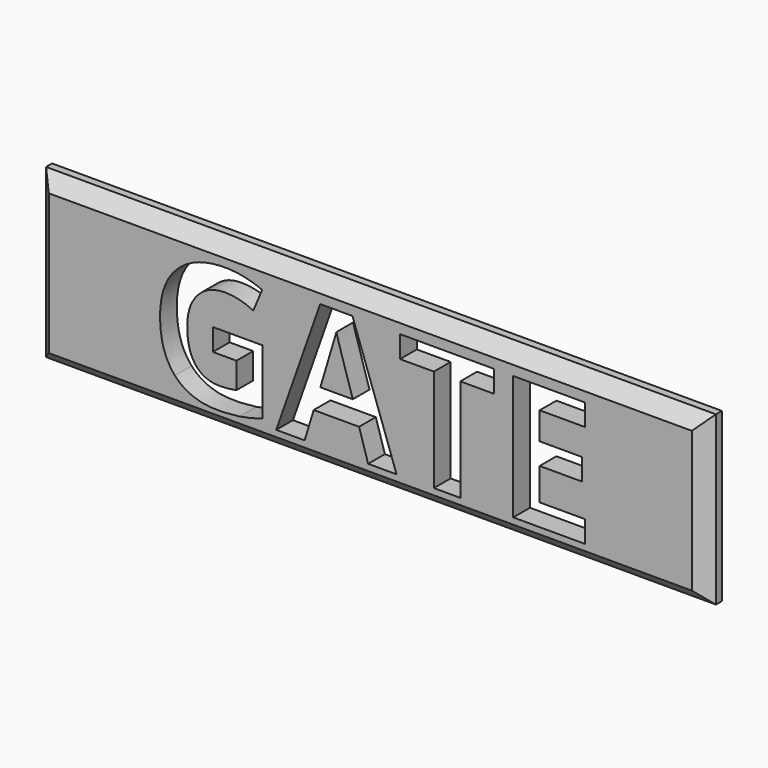
from build123d import *

# Parameters (mm, degrees)
F0_W     = 50.8
F0_H     = 12.7
F1_DEPTH = 1.5875
F2_SIZE  = 1.016


# Not quite as in the source:
# - a feature names something its author has since deleted; it is built from what else it names


with BuildPart() as f1:
    # F0 (on Front) → F1 (new body)
    with BuildSketch(Plane.XZ):
        with Locations((-9.1615320603, 10.3311909613)):
            Rectangle(F0_W, F0_H)
        with BuildLine():
            Line((-21.1010067493, 9.1154048977), (-21.1010067493, 10.7835201321))
            Line((-21.1010067493, 10.7835201321), (-17.3534318796, 10.7835201321))
            Line((-17.3534318796, 10.7835201321), (-17.3534318796, 5.8866614081))
            add(Edge.make_bspline(
                [(-17.3534318796, 5.8866614081), (-18.2650041452, 5.5890051581), (-19.0690894316, 5.4691158352)],
                knots=[0, 0, 0, 1, 1, 1], degree=2))
            add(Edge.make_bspline(
                [(-19.0690894316, 5.4691158352), (-19.8731747181, 5.3492265123), (-20.7123999785, 5.3492265123)],
                knots=[0, 0, 0, 1, 1, 1], degree=2))
            add(Edge.make_bspline(
                [(-20.7123999785, 5.3492265123), (-22.8497372181, 5.3492265123), (-23.9773169707, 6.6059973456)],
                knots=[0, 0, 0, 1, 1, 1], degree=2))
            add(Edge.make_bspline(
                [(-23.9773169707, 6.6059973456), (-25.1048967233, 7.862768179), (-25.1048967233, 10.2150793769)],
                knots=[0, 0, 0, 1, 1, 1], degree=2))
            add(Edge.make_bspline(
                [(-25.1048967233, 10.2150793769), (-25.1048967233, 12.5012447415), (-23.7964494577, 13.7797196764)],
                knots=[0, 0, 0, 1, 1, 1], degree=2))
            add(Edge.make_bspline(
                [(-23.7964494577, 13.7797196764), (-22.4880021921, 15.0581946113), (-20.1708309681, 15.0581946113)],
                knots=[0, 0, 0, 1, 1, 1], degree=2))
            add(Edge.make_bspline(
                [(-20.1708309681, 15.0581946113), (-18.7156226348, 15.0581946113), (-17.3658342233, 14.4773515123)],
                knots=[0, 0, 0, 1, 1, 1], degree=2))
            Line((-17.3658342233, 14.4773515123), (-18.0314266712, 12.8753821113))
            add(Edge.make_bspline(
                [(-18.0314266712, 12.8753821113), (-19.0649553171, 13.3921464342), (-20.1832333118, 13.3921464342)],
                knots=[0, 0, 0, 1, 1, 1], degree=2))
            add(Edge.make_bspline(
                [(-20.1832333118, 13.3921464342), (-21.481345291, 13.3921464342), (-22.2626929473, 12.5198482571)],
                knots=[0, 0, 0, 1, 1, 1], degree=2))
            add(Edge.make_bspline(
                [(-22.2626929473, 12.5198482571), (-23.0440406035, 11.64755008), (-23.0440406035, 10.1758052883)],
                knots=[0, 0, 0, 1, 1, 1], degree=2))
            add(Edge.make_bspline(
                [(-23.0440406035, 10.1758052883), (-23.0440406035, 8.6379146633), (-22.4146216582, 7.827628205)],
                knots=[0, 0, 0, 1, 1, 1], degree=2))
            add(Edge.make_bspline(
                [(-22.4146216582, 7.827628205), (-21.7852027129, 7.0173417467), (-20.5842424264, 7.0173417467)],
                knots=[0, 0, 0, 1, 1, 1], degree=2))
            add(Edge.make_bspline(
                [(-20.5842424264, 7.0173417467), (-19.9558570098, 7.0173417467), (-19.3109351348, 7.1454992988)],
                knots=[0, 0, 0, 1, 1, 1], degree=2))
            Line((-19.3109351348, 7.1454992988), (-19.3109351348, 9.1154048977))
            Line((-19.3109351348, 9.1154048977), (-21.1010067493, 9.1154048977))
        make_face(mode=Mode.SUBTRACT)
        Polygon((-7.1669735462, 5.4794511217), (-9.3249813587, 5.4794511217), (-10.0091773223, 7.728409455), (-13.4528947702, 7.728409455), (-14.1370907337, 5.4794511217), (-16.2950985462, 5.4794511217), (-12.9609351348, 14.9631099758), (-10.5135393014, 14.9631099758), align=None, mode=Mode.SUBTRACT)
        Polygon((-2.3341935983, 13.2577877102), (-2.3341935983, 5.4794511217), (-4.3371721139, 5.4794511217), (-4.3371721139, 13.2577877102), (-6.9023902129, 13.2577877102), (-6.9023902129, 14.9238358873), (0.2289574434, 14.9238358873), (0.2289574434, 13.2577877102), align=None, mode=Mode.SUBTRACT)
        Polygon((7.1205264538, 7.133096955), (7.1205264538, 5.4794511217), (1.6820987194, 5.4794511217), (1.6820987194, 14.9238358873), (7.1205264538, 14.9238358873), (7.1205264538, 13.2825923977), (3.685077235, 13.2825923977), (3.685077235, 11.2093339342), (6.8828148652, 11.2093339342), (6.8828148652, 9.5680904446), (3.685077235, 9.5680904446), (3.685077235, 7.133096955), align=None, mode=Mode.SUBTRACT)
    extrude(amount=F1_DEPTH)

    # F2
    f2_edges = [f1.edges().sort_by_distance(p)[0] for p in [
        (-9.161532, -1.5875, 3.981191),
        (-34.561532, -1.5875, 10.331191),
        (-9.161532, -1.5875, 16.681191),
        (16.238468, -1.5875, 10.331191),
    ]]
    chamfer(f2_edges, length=F2_SIZE)


with BuildPart() as f1b:
    # F0 (on Front) → F1, piece 2 (new body)
    with BuildSketch(Plane.XZ):
        with BuildLine():
            Line((-12.948532791, 9.4068599758), (-10.4887346139, 9.4068599758))
            add(Edge.make_bspline(
                [(-10.4887346139, 9.4068599758), (-11.4375139108, 12.4619706529), (-11.5574032337, 12.8629797675)],
                knots=[0, 0, 0, 1, 1, 1], degree=2))
            add(Edge.make_bspline(
                [(-11.5574032337, 12.8629797675), (-11.6772925566, 13.2639888821), (-11.7289689889, 13.4954992988)],
                knots=[0, 0, 0, 1, 1, 1], degree=2))
            add(Edge.make_bspline(
                [(-11.7289689889, 13.4954992988), (-11.94187589, 12.6686763821), (-12.948532791, 9.4068599758)],
                knots=[0, 0, 0, 1, 1, 1], degree=2))
        make_face()
    extrude(amount=F1_DEPTH)


solid = Compound([f1.part, f1b.part])
